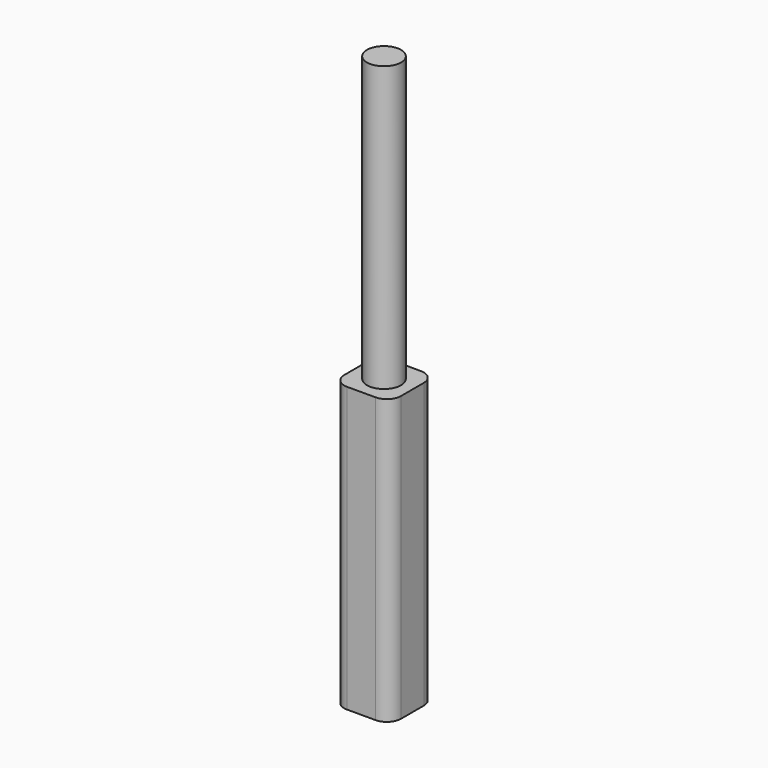
from build123d import *

# Parameters (mm, degrees)
F0_R     = 6
F1_DEPTH = 100
F3_DEPTH = 100


with BuildPart() as f1:
    # F0 (on Top) → F1 (new body)
    with BuildSketch(Plane.XY):
        Circle(F0_R)
    extrude(amount=F1_DEPTH)

    # F2 (on face) → F3 (join)
    with BuildSketch(Plane(origin=(0, 0, 0), x_dir=(1, 0, 0), z_dir=(0, 0, -1))):
        with BuildLine():
            ThreePointArc((0, -6), (-4.2426406871, -4.2426406871), (-6, 0))
            Line((-6, 0), (-10, 0))
            Line((-10, 0), (-10, -5))
            ThreePointArc((-10, -5), (-8.5355339059, -8.5355339059), (-5, -10))
            Line((-5, -10), (0, -10))
            Line((0, -10), (0, -6))
        make_face()
        with BuildLine():
            Line((-10, 0), (-6, 0))
            ThreePointArc((-6, 0), (-4.2426406871, 4.2426406871), (0, 6))
            Line((0, 6), (0, 10))
            Line((0, 10), (-5, 10))
            ThreePointArc((-5, 10), (-8.5355339059, 8.5355339059), (-10, 5))
            Line((-10, 5), (-10, 0))
        make_face()
        with BuildLine():
            ThreePointArc((0, 6), (-4.2426406871, 4.2426406871), (-6, 0))
            ThreePointArc((-6, 0), (-4.2426406871, -4.2426406871), (0, -6))
            ThreePointArc((0, -6), (4.2426406871, -4.2426406871), (6, 0))
            ThreePointArc((6, 0), (4.2426406871, 4.2426406871), (0, 6))
        make_face()
        with BuildLine():
            Line((0, 10), (0, 6))
            ThreePointArc((0, 6), (4.2426406871, 4.2426406871), (6, 0))
            Line((6, 0), (10, 0))
            Line((10, 0), (10, 5))
            ThreePointArc((10, 5), (8.5355339059, 8.5355339059), (5, 10))
            Line((5, 10), (0, 10))
        make_face()
        with BuildLine():
            ThreePointArc((6, 0), (4.2426406871, -4.2426406871), (0, -6))
            Line((0, -6), (0, -10))
            Line((0, -10), (5, -10))
            ThreePointArc((5, -10), (8.5355339059, -8.5355339059), (10, -5))
            Line((10, -5), (10, 0))
            Line((10, 0), (6, 0))
        make_face()
    extrude(amount=F3_DEPTH)


solid = f1.part
